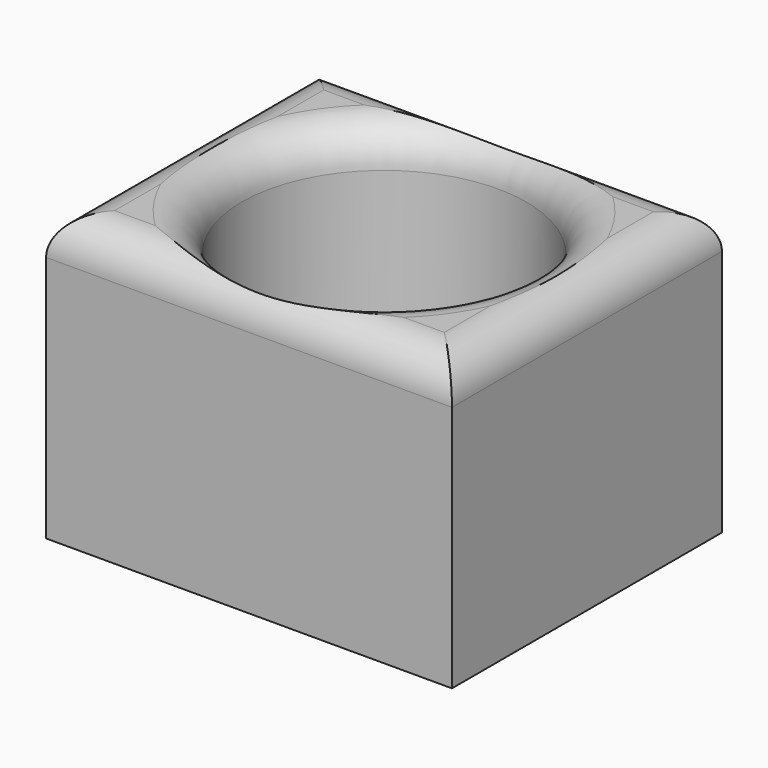
from build123d import *

# Parameters (mm, degrees)
F0_W        = 108.3307564259
F0_H        = 90.0692865252
F0_R        = 37.9662670308
F1_DEPTH    = 76.2
F2_T1_DEPTH = 159.1307564259
F2_T3_DEPTH = 140.8692865252


# Not quite as in the source:
# - a fillet or chamfer that OpenCascade refuses, or shapes differently, is made with other operations: its cross-section is extruded or revolved along the edge and cut away or added


with BuildPart() as f1:
    # F0 (on Top) → F1 (new body)
    with BuildSketch(Plane.XY):
        Rectangle(F0_W, F0_H)
        Circle(F0_R, mode=Mode.SUBTRACT)
    extrude(amount=F1_DEPTH)

    # F2: fillet of radius 10.16 on 5 edges, made by hand

    # F2_s2 → F2_t1 (cut)
    with BuildSketch(Plane.YZ.offset(-79.5653782129)):
        with BuildLine():
            ThreePointArc((-45.0346432626, 66.04), (-42.0588481595, 73.2242048969), (-34.8746432626, 76.2))
            Line((-34.8746432626, 76.2), (-45.0346432626, 76.2))
            Line((-45.0346432626, 76.2), (-45.0346432626, 66.04))
        make_face()
        with BuildLine():
            ThreePointArc((45.0346432626, 66.04), (42.0588481595, 73.2242048969), (34.8746432626, 76.2))
            Line((34.8746432626, 76.2), (45.0346432626, 76.2))
            Line((45.0346432626, 76.2), (45.0346432626, 66.04))
        make_face()
    extrude(amount=F2_T1_DEPTH, mode=Mode.SUBTRACT)

    # F2_s4 → F2_t3 (cut)
    with BuildSketch(Plane.XZ.offset(-70.4346432626)):
        with BuildLine():
            ThreePointArc((-54.1653782129, 66.04), (-51.1895831098, 73.2242048969), (-44.0053782129, 76.2))
            Line((-44.0053782129, 76.2), (-54.1653782129, 76.2))
            Line((-54.1653782129, 76.2), (-54.1653782129, 66.04))
        make_face()
        with BuildLine():
            ThreePointArc((54.1653782129, 66.04), (51.1895831098, 73.2242048969), (44.0053782129, 76.2))
            Line((44.0053782129, 76.2), (54.1653782129, 76.2))
            Line((54.1653782129, 76.2), (54.1653782129, 66.04))
        make_face()
    extrude(amount=F2_T3_DEPTH, mode=Mode.SUBTRACT)

    # F2_s5 → F2_t6 (revolve, cut)
    with BuildSketch(Plane.XZ):
        with BuildLine():
            ThreePointArc((37.9662670308, 66.04), (40.9420621339, 73.2242048969), (48.1262670308, 76.2))
            Line((48.1262670308, 76.2), (37.9662670308, 76.2))
            Line((37.9662670308, 76.2), (37.9662670308, 66.04))
        make_face()
    revolve(axis=Axis((0, 0, 76.2), (0, 0, 1)), mode=Mode.SUBTRACT)


solid = f1.part
